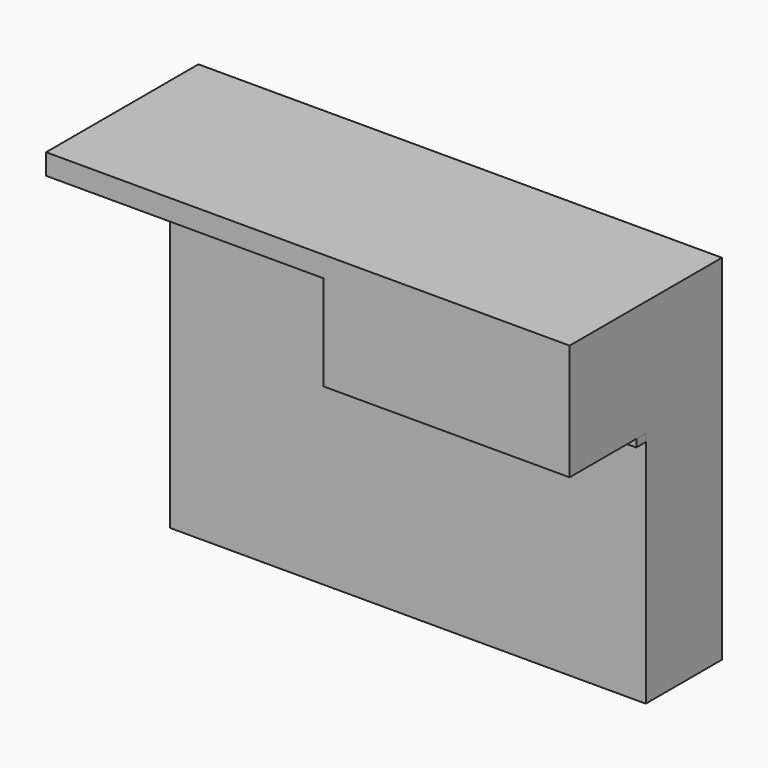
from build123d import *

# Parameters (mm, degrees)
F0_W          = 482.8630983498
F0_H          = 200
F1_DEPTH      = 200
F0_H_2        = 43.6560429633
F2_DEPTH      = 200
F2_DEPTH_BACK = 200
F3_W          = 501.3401806686
F3_H          = 16
F4_DEPTH      = 25
F3_W_2        = 422.7913618088
F3_W_3        = 16
F3_H_2        = 143.8153088093
F3_W_4        = 15.9996449616
F5_DEPTH      = 25
F6_W          = 400
F6_H          = 43.6560429633
F7_DEPTH      = 100
F8_W          = 20.3876569867
F8_H          = 16
F5_FACE_W     = 25
F5_FACE_H     = 16
F9_DEPTH      = 25
F8_W_2        = 179.6123430133
F10_DEPTH     = 25


with BuildPart() as f1:
    # F0 (on Front) → F1 (new body)
    with BuildSketch(Plane.XZ):
        Polygon((-192.7827596664, 248.3553551137), (-675.6458580162, 248.3553551137), (-675.6458580162, -251.6446448863), (324.3541419838, -251.6446448863), (324.3541419838, 248.3553551137), align=None)
        with Locations((-434.2143088413, 348.3553551137)):
            Rectangle(F0_W, F0_H)
    extrude(amount=-F1_DEPTH)

    # F0 (on Front) → F2 (join, two sides)
    with BuildSketch(Plane.XZ) as f2_sk:
        with Locations((-434.2143088413, 470.1833765954)):
            Rectangle(F0_W, F0_H_2)
        Polygon((-192.7827596664, 448.3553551137), (-192.7827596664, 248.3553551137), (324.3541419838, 248.3553551137), (324.3541419838, 492.011398077), (-192.7827596664, 492.011398077), align=None)
    extrude(amount=F2_DEPTH)
    extrude(f2_sk.sketch, amount=-F2_DEPTH_BACK)

    # F6 (on face) → F7 (join)
    with BuildSketch(Plane(origin=(-675.6458580162, 0, 0), x_dir=(0, -1, 0), z_dir=(-1, 0, 0))):
        with Locations((0, 470.1833765954)):
            Rectangle(F6_W, F6_H)
    extrude(amount=F7_DEPTH)


with BuildPart() as f4:
    # F3 (on face) → F4 (new body)
    with BuildSketch(Plane.XZ):
        with Locations((73.6840516495, 240.3553551137)):
            Rectangle(F3_W, F3_H)
    extrude(amount=F4_DEPTH)


with BuildPart() as f4b:
    # F3 (on face) → F4, piece 2 (new body)
    with BuildSketch(Plane.XZ):
        with Locations((-448.2505321503, 440.3553551137)):
            Rectangle(F3_W_2, F3_H)
    extrude(amount=F4_DEPTH)


with BuildPart() as f4c:
    # F3 (on face) → F4, piece 3 (new body)
    with BuildSketch(Plane.XZ):
        with Locations((-200.7827596664, 333.9206725359)):
            Rectangle(F3_W_3, F3_H_2)
    extrude(amount=F4_DEPTH)


with BuildPart() as f5:
    # F3 (on face) → F5 (new body)
    with BuildSketch(Plane.XZ):
        with Locations((-667.6460355355, 440.3553551137)):
            Rectangle(F3_W_4, F3_H)
    extrude(amount=F5_DEPTH)

    # F8 (on face) + F5_face (on face) → F9 (join)
    with BuildSketch(Plane(origin=(-675.6458580162, 0, 0), x_dir=(0, -1, 0), z_dir=(-1, 0, 0))):
        with Locations((-10.1938284934, 440.3553551137)):
            Rectangle(F8_W, F8_H)
    with BuildSketch(Plane(origin=(-675.6458580162, -12.5, 440.3553551137), x_dir=(0, -1, 0), z_dir=(-1, 0, 0))):
        Rectangle(F5_FACE_W, F5_FACE_H)
    extrude(amount=F9_DEPTH)


with BuildPart() as f5b:
    # F3 (on face) → F5, piece 2 (new body)
    with BuildSketch(Plane.XZ):
        Polygon((-192.7827596664, 448.3553551137), (-236.8548512459, 448.3553551137), (-236.8548512459, 432.3553551137), (-208.7827596664, 432.3553551137), (-208.7827596664, 405.8283269405), (-192.7827596664, 405.8283269405), (-192.7827596664, 423.3553551137), (-192.7827596664, 432.3553551137), align=None)
    extrude(amount=F5_DEPTH)


with BuildPart() as f5c:
    # F3 (on face) → F5, piece 3 (new body)
    with BuildSketch(Plane.XZ):
        Polygon((-192.7827596664, 232.3553551137), (-176.9860386848, 232.3553551137), (-176.9860386848, 248.3553551137), (-192.7827596664, 248.3553551137), (-192.7827596664, 262.0130181313), (-208.7827596664, 262.0130181313), (-208.7827596664, 232.3553551137), align=None)
    extrude(amount=F5_DEPTH)


with BuildPart() as f10:
    # F8 (on face) → F10 (new body)
    with BuildSketch(Plane(origin=(-675.6458580162, 0, 0), x_dir=(0, -1, 0), z_dir=(-1, 0, 0))):
        with Locations((-110.1938284934, 440.3553551137)):
            Rectangle(F8_W_2, F8_H)
    extrude(amount=F10_DEPTH)


solid = Compound([f1.part, f4.part, f4b.part, f4c.part, f5.part, f5b.part, f5c.part, f10.part])
